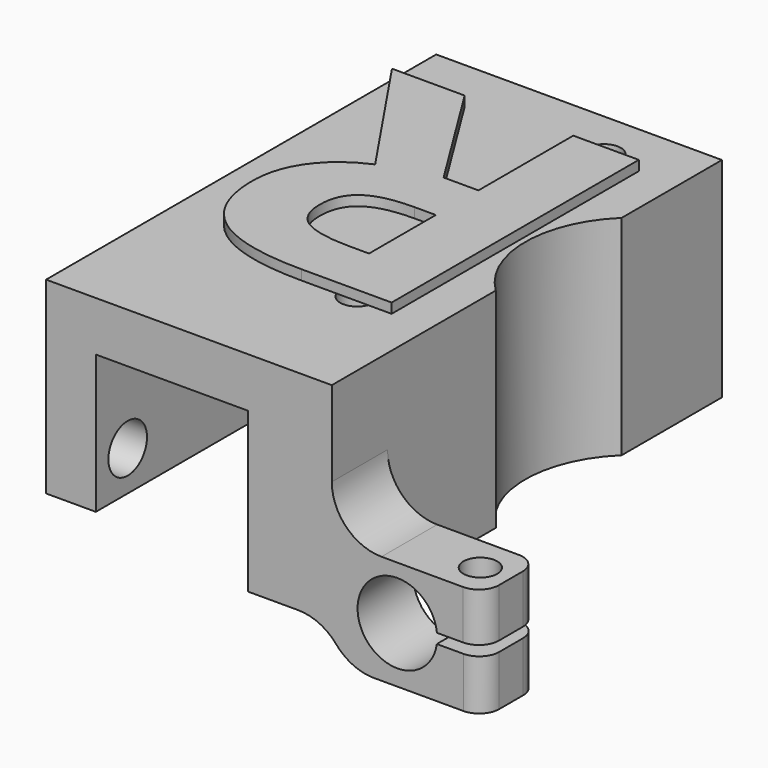
from build123d import *

# Parameters (mm, degrees)
F1_DEPTH      = 7
F2_DEPTH      = 42
F3_R          = 1.7
F3_R_2        = 11
F4_DEPTH      = 21.001
F5_R          = 4
F6_DEPTH      = 10
F7_DEPTH      = 21.001
F8_R          = 1.4
F9_DEPTH      = 11.0256338484
F8_R_2        = 1.7
F10_DEPTH     = 4.9110969969
F11_R         = 5
F12_R         = 5
F13_R         = 5
F14_R         = 2
F15_R         = 2.2
F15_R_2       = 2.4255023423
F16_DEPTH     = 6
F17_TEXT_SIZE = 43.4899399227
F18_DEPTH     = 1


# Not quite as in the source:
# - a feature names something its author has since deleted; it is built from what else it names
# - Text() gives the source's letters only with a copy of the font that has no kerning and outlines rounded to 1/6400 em; it was checked with that copy


with BuildPart() as f1:
    # F0 (on Front) → F1 (new body)
    with BuildSketch(Plane.XZ):
        Polygon((-18.6721007523, 29.8099789735), (-18.6721007523, 10.8925135386), (-13.6721007523, 10.8925135386), (-13.6721007523, 24.8099789735), (1.6278992477, 24.8099789735), (1.6278992477, 8.8099789735), (10.0380548998, 8.8099789735), (10.0380548998, 16.2656020473), (10.0380548998, 29.8099789735), align=None)
        Polygon((25.2263195603, 16.2417280634), (10.0380548998, 16.2656020473), (10.0380548998, 8.8099789735), (11.4533044869, 5.2860832236), (25.2553367778, 5.2860832236), (25.2553367778, 10.343908232), (18.5860510706, 10.343908232), (18.5860510706, 11.3388913612), (25.2263195603, 11.3388913612), align=None)
    extrude(amount=F1_DEPTH)

    # F0 (on Front) → F2 (join)
    with BuildSketch(Plane.XZ):
        Polygon((-18.6721007523, 29.8099789735), (-18.6721007523, 10.8925135386), (-13.6721007523, 10.8925135386), (-13.6721007523, 24.8099789735), (1.6278992477, 24.8099789735), (1.6278992477, 8.8099789735), (10.0380548998, 8.8099789735), (10.0380548998, 16.2656020473), (10.0380548998, 29.8099789735), align=None)
    extrude(amount=-F2_DEPTH)

    # F3 (on face) → F4 (cut, through all)
    with BuildSketch(Plane(origin=(0, 0, 8.8099789735), x_dir=(1, 0, 0), z_dir=(0, 0, -1))):
        with Locations((2.1850741468, -6)):
            Circle(F3_R)
        with Locations((2.1850741468, -37)):
            Circle(F3_R)
        with Locations((17.6850741468, -21.5)):
            Circle(F3_R_2)
    extrude(amount=-F4_DEPTH, mode=Mode.SUBTRACT)

    # F5 (on face) → F6 (cut)
    with BuildSketch(Plane.XZ.offset(7)):
        with Locations((16.6278992477, 10.8989789735)):
            Circle(F5_R)
    extrude(amount=-F6_DEPTH, mode=Mode.SUBTRACT)

    # F3 (on face) → F7 (cut, through all)
    with BuildSketch(Plane(origin=(0, 0, 8.8099789735), x_dir=(1, 0, 0), z_dir=(0, 0, -1))):
        with Locations((2.1850741468, -6)):
            Circle(F3_R)
        with Locations((2.1850741468, -37)):
            Circle(F3_R)
        with Locations((17.6850741468, -21.5)):
            Circle(F3_R_2)
    extrude(amount=-F7_DEPTH, mode=Mode.SUBTRACT)

    # F8 (on face) → F9 (cut, through all)
    with BuildSketch(Plane(origin=(0.0255921572, 0, 16.2813403413), x_dir=(0.9999987646, 0, -0.0015718685), z_dir=(0.0015718685, 0, 0.9999987646))):
        with Locations((22.2007585357, -3.5767070949)):
            Circle(F8_R)
    extrude(amount=-F9_DEPTH, mode=Mode.SUBTRACT)

    # F8 (on face) → F10 (cut, through all)
    with BuildSketch(Plane(origin=(0.0255921572, 0, 16.2813403413), x_dir=(0.9999987646, 0, -0.0015718685), z_dir=(0.0015718685, 0, 0.9999987646))):
        with Locations((22.2007585357, -3.5767070949)):
            Circle(F8_R_2)
        with Locations((22.2007585357, -3.5767070949)):
            Circle(F8_R, mode=Mode.SUBTRACT)
    extrude(amount=-F10_DEPTH, mode=Mode.SUBTRACT)

    # F11
    f11_edges = [f1.edges().sort_by_distance(p)[0] for p in [
        (10.038055, -3.5, 16.265602),
    ]]
    fillet(f11_edges, radius=F11_R)

    # F12
    f12_edges = [f1.edges().sort_by_distance(p)[0] for p in [
        (10.038055, -3.5, 8.809979),
    ]]
    fillet(f12_edges, radius=F12_R)

    # F13
    f13_edges = [f1.edges().sort_by_distance(p)[0] for p in [
        (11.453304, -3.5, 5.286083),
    ]]
    fillet(f13_edges, radius=F13_R)

    # F14
    f14_edges = [f1.edges().sort_by_distance(p)[0] for p in [
        (25.22632, -7, 13.79031),
        (25.255337, -7, 7.814996),
        (25.22632, 0, 13.79031),
        (25.255337, 0, 7.814996),
    ]]
    fillet(f14_edges, radius=F14_R)

    # F15 (on face) → F16 (cut)
    with BuildSketch(Plane(origin=(-18.6721007523, 0, 0), x_dir=(0, -1, 0), z_dir=(-1, 0, 0))):
        with Locations((-38, 14.8925135386)):
            Circle(F15_R)
        with Locations((3, 14.8925135386)):
            Circle(F15_R_2)
    extrude(amount=-F16_DEPTH, mode=Mode.SUBTRACT)

    # F17 (on face) → F18 (join)
    with BuildSketch(Plane.XY.offset(29.8099789735)):
        with Locations(Location((10.0380548998, 36.4449019432), (0, 0, 180))):
            Text('R', F17_TEXT_SIZE, font='Open Sans', font_style=FontStyle.BOLD, text_align=(TextAlign.LEFT, TextAlign.BOTTOM))
    extrude(amount=F18_DEPTH)


solid = f1.part
